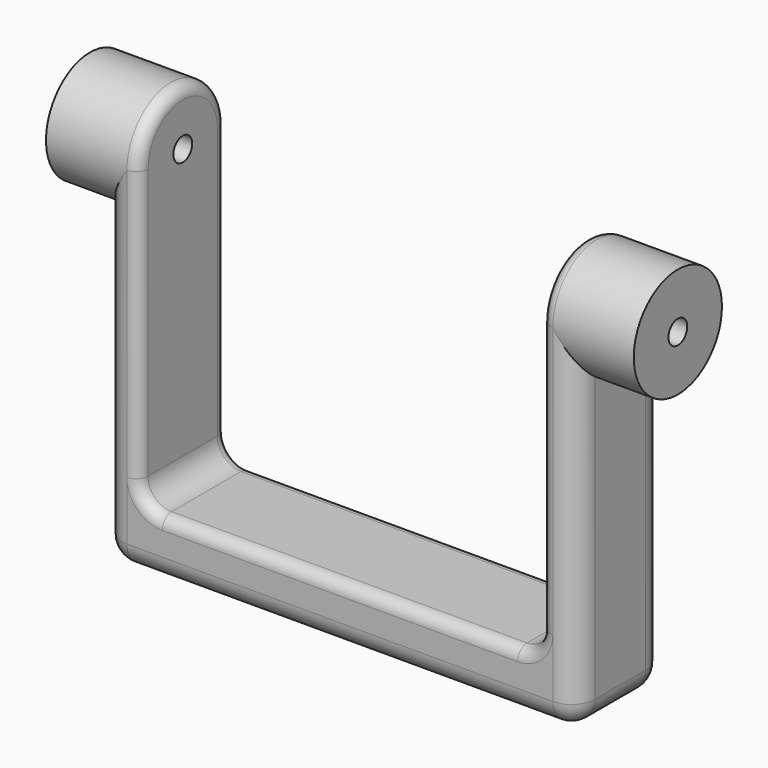
from build123d import *

# Parameters (mm, degrees)
F0_W          = 102.1880283952
F0_H          = 23.8108858466
F1_DEPTH      = 38.1
F2_R          = 11.9054429233
F3_DEPTH      = 63.5
F4_W          = 86.9480283952
F4_H          = 88.2315921943
F5_DEPTH      = 25.4
F6_R          = 2.54
F7_DEPTH      = 63.5
F8_T1_DEPTH   = 127.5880283952
F8_T6_DEPTH   = 101.6
F8_S7_R       = 11.9054429233
F8_T8_DEPTH   = 52
F8_T12_DEPTH  = 101.6
F8_S13_R      = 11.9054429233
F8_T14_DEPTH  = 52
F9_T1_DEPTH   = 127.5880283952
F9_T6_DEPTH   = 101.6
F9_S7_R       = 11.9054429233
F9_T8_DEPTH   = 52
F9_T12_DEPTH  = 101.6
F9_S13_R      = 11.9054429233
F9_T14_DEPTH  = 52
F10_T1_DEPTH  = 13.6508858466
F10_S5_W      = 5.08
F10_S5_H      = 5.08
F10_T6_DEPTH  = 5.08
F10_S11_W     = 5.08
F10_S11_H     = 5.08
F10_T12_DEPTH = 5.08
F10_S17_W     = 5.08
F10_S17_H     = 5.08
F10_T18_DEPTH = 5.08
F10_S23_W     = 5.08
F10_S23_H     = 5.08
F10_T24_DEPTH = 5.08
F11_R         = 5.08
F12_R         = 2.53999


# Not quite as in the source:
# - a fillet or chamfer that OpenCascade refuses, or shapes differently, is made with other operations: its cross-section is extruded or revolved along the edge and cut away or added
# - a fillet or chamfer is up to 0.001 mm smaller than in the source, because OpenCascade refuses the exact size


with BuildPart() as f1:
    # F0 (on Top) → F1 (new body, symmetric)
    with BuildSketch(Plane.XY):
        Rectangle(F0_W, F0_H)
    extrude(amount=F1_DEPTH, both=True)

    # F2 (on Right) → F3 (join, symmetric)
    with BuildSketch(Plane.YZ):
        with Locations((0, 38.1)):
            Circle(F2_R)
    extrude(amount=F3_DEPTH, both=True)

    # F4 (on Front) → F5 (cut, symmetric)
    with BuildSketch(Plane.XZ):
        with Locations((0, 18.7157960971)):
            Rectangle(F4_W, F4_H)
    extrude(amount=F5_DEPTH, both=True, mode=Mode.SUBTRACT)

    # F6 (on Right) → F7 (cut, symmetric)
    with BuildSketch(Plane.YZ):
        with Locations((0, 38.1)):
            Circle(F6_R)
    extrude(amount=F7_DEPTH, both=True, mode=Mode.SUBTRACT)

    # F8: fillet of radius 5.08 on 3 edges, made by hand

    # F8_s2 → F8_t1 (cut)
    with BuildSketch(Plane.YZ.offset(-63.7940141976)):
        with BuildLine():
            ThreePointArc((-6.8254429233, -38.1), (-10.4175453717, -36.6121024484), (-11.9054429233, -33.02))
            Line((-11.9054429233, -33.02), (-11.9054429233, -38.1))
            Line((-11.9054429233, -38.1), (-6.8254429233, -38.1))
        make_face()
    extrude(amount=F8_T1_DEPTH, mode=Mode.SUBTRACT)


with BuildPart() as f8_tool4:
    # F8_s5 → F8_t6 (new body)
    with BuildSketch(Plane.XY.offset(50.8)):
        with BuildLine():
            ThreePointArc((51.0940141976, -6.8254429233), (49.606116646, -10.4175453717), (46.0140141976, -11.9054429233))
            Line((46.0140141976, -11.9054429233), (51.0940141976, -11.9054429233))
            Line((51.0940141976, -11.9054429233), (51.0940141976, -6.8254429233))
        make_face()
    extrude(amount=-F8_T6_DEPTH)

    # F8_s7 → F8_t8 (cut, symmetric)
    with BuildSketch(Plane.YZ.offset(48.6)):
        with Locations((0, 38.1)):
            Circle(F8_S7_R)
    extrude(amount=F8_T8_DEPTH, both=True, mode=Mode.SUBTRACT)


with BuildPart() as f1_1:
    add(f1.part)

    # F8_t3: cut F8_tool4
    add(f8_tool4.part, mode=Mode.SUBTRACT)


with BuildPart() as f8_tool10:
    # F8_s11 → F8_t12 (new body)
    with BuildSketch(Plane.XY.offset(-50.8)):
        with BuildLine():
            ThreePointArc((-51.0940141976, -6.8254429233), (-49.606116646, -10.4175453717), (-46.0140141976, -11.9054429233))
            Line((-46.0140141976, -11.9054429233), (-51.0940141976, -11.9054429233))
            Line((-51.0940141976, -11.9054429233), (-51.0940141976, -6.8254429233))
        make_face()
    extrude(amount=F8_T12_DEPTH)

    # F8_s13 → F8_t14 (cut, symmetric)
    with BuildSketch(Plane.YZ.offset(-48.6)):
        with Locations((0, 38.1)):
            Circle(F8_S13_R)
    extrude(amount=F8_T14_DEPTH, both=True, mode=Mode.SUBTRACT)


with BuildPart() as f1_2:
    add(f1_1.part)

    # F8_t9: cut F8_tool10
    add(f8_tool10.part, mode=Mode.SUBTRACT)

    # F9: fillet of radius 5.08 on 3 edges, made by hand

    # F9_s2 → F9_t1 (cut)
    with BuildSketch(Plane.YZ.offset(-63.7940141976)):
        with BuildLine():
            ThreePointArc((11.9054429233, -33.02), (10.4175453717, -36.6121024484), (6.8254429233, -38.1))
            Line((6.8254429233, -38.1), (11.9054429233, -38.1))
            Line((11.9054429233, -38.1), (11.9054429233, -33.02))
        make_face()
    extrude(amount=F9_T1_DEPTH, mode=Mode.SUBTRACT)


with BuildPart() as f9_tool4:
    # F9_s5 → F9_t6 (new body)
    with BuildSketch(Plane.XY.offset(-50.8)):
        with BuildLine():
            ThreePointArc((-46.0140141976, 11.9054429233), (-49.606116646, 10.4175453717), (-51.0940141976, 6.8254429233))
            Line((-51.0940141976, 6.8254429233), (-51.0940141976, 11.9054429233))
            Line((-51.0940141976, 11.9054429233), (-46.0140141976, 11.9054429233))
        make_face()
    extrude(amount=F9_T6_DEPTH)

    # F9_s7 → F9_t8 (cut, symmetric)
    with BuildSketch(Plane.YZ.offset(-48.6)):
        with Locations((0, 38.1)):
            Circle(F9_S7_R)
    extrude(amount=F9_T8_DEPTH, both=True, mode=Mode.SUBTRACT)


with BuildPart() as f1_3:
    add(f1_2.part)

    # F9_t3: cut F9_tool4
    add(f9_tool4.part, mode=Mode.SUBTRACT)


with BuildPart() as f9_tool10:
    # F9_s11 → F9_t12 (new body)
    with BuildSketch(Plane.XY.offset(50.8)):
        with BuildLine():
            ThreePointArc((46.0140141976, 11.9054429233), (49.606116646, 10.4175453717), (51.0940141976, 6.8254429233))
            Line((51.0940141976, 6.8254429233), (51.0940141976, 11.9054429233))
            Line((51.0940141976, 11.9054429233), (46.0140141976, 11.9054429233))
        make_face()
    extrude(amount=-F9_T12_DEPTH)

    # F9_s13 → F9_t14 (cut, symmetric)
    with BuildSketch(Plane.YZ.offset(48.6)):
        with Locations((0, 38.1)):
            Circle(F9_S13_R)
    extrude(amount=F9_T14_DEPTH, both=True, mode=Mode.SUBTRACT)


with BuildPart() as f1_4:
    add(f1_3.part)

    # F9_t9: cut F9_tool10
    add(f9_tool10.part, mode=Mode.SUBTRACT)

    # F10: fillet of radius 5.08 on 2 edges, made by hand

    # F10_s2 → F10_t1 (cut)
    with BuildSketch(Plane.XZ.offset(-6.8254429233)):
        with BuildLine():
            ThreePointArc((-46.0140141976, -38.1), (-49.606116646, -36.6121024484), (-51.0940141976, -33.02))
            Line((-51.0940141976, -33.02), (-51.0940141976, -38.1))
            Line((-51.0940141976, -38.1), (-46.0140141976, -38.1))
        make_face()
        with BuildLine():
            ThreePointArc((46.0140141976, -38.1), (49.606116646, -36.6121024484), (51.0940141976, -33.02))
            Line((51.0940141976, -33.02), (51.0940141976, -38.1))
            Line((51.0940141976, -38.1), (46.0140141976, -38.1))
        make_face()
    extrude(amount=F10_T1_DEPTH, mode=Mode.SUBTRACT)


with BuildPart() as f10_tool4:
    # F10_s5 → F10_t6 (new body)
    with BuildSketch(Plane.XY.offset(-33.02)):
        with Locations((48.5540141976, -9.3654429233)):
            Rectangle(F10_S5_W, F10_S5_H)
    extrude(amount=-F10_T6_DEPTH)

    # F10_s7 → F10_t8 (revolve, cut)
    with BuildSketch(Plane(origin=(46.0140141976, -6.8254429233, -33.02), x_dir=(-0.7071067812, 0.7071067812, 0), z_dir=(-0.7071067812, -0.7071067812, 0))):
        with BuildLine():
            ThreePointArc((0, -5.08), (5.08, 0), (0, 5.08))
            Line((0, 5.08), (0, -5.08))
        make_face()
    revolve(axis=Axis((46.0140141976, -6.8254429233, -33.02), (0, 0, -1)), mode=Mode.SUBTRACT)


with BuildPart() as f1_5:
    add(f1_4.part)

    # F10_t3: cut F10_tool4
    add(f10_tool4.part, mode=Mode.SUBTRACT)


with BuildPart() as f10_tool10:
    # F10_s11 → F10_t12 (new body)
    with BuildSketch(Plane.XY.offset(-33.02)):
        with Locations((48.5540141976, 9.3654429233)):
            Rectangle(F10_S11_W, F10_S11_H)
    extrude(amount=-F10_T12_DEPTH)

    # F10_s13 → F10_t14 (revolve, cut)
    with BuildSketch(Plane(origin=(46.0140141976, 6.8254429233, -33.02), x_dir=(-0.7071067812, -0.7071067812, 0), z_dir=(0.7071067812, -0.7071067812, 0))):
        with BuildLine():
            ThreePointArc((0, -5.08), (5.08, 0), (0, 5.08))
            Line((0, 5.08), (0, -5.08))
        make_face()
    revolve(axis=Axis((46.0140141976, 6.8254429233, -33.02), (0, 0, -1)), mode=Mode.SUBTRACT)


with BuildPart() as f1_6:
    add(f1_5.part)

    # F10_t9: cut F10_tool10
    add(f10_tool10.part, mode=Mode.SUBTRACT)


with BuildPart() as f10_tool16:
    # F10_s17 → F10_t18 (new body)
    with BuildSketch(Plane.XY.offset(-33.02)):
        with Locations((-48.5540141976, 9.3654429233)):
            Rectangle(F10_S17_W, F10_S17_H)
    extrude(amount=-F10_T18_DEPTH)

    # F10_s19 → F10_t20 (revolve, cut)
    with BuildSketch(Plane(origin=(-46.0140141976, 6.8254429233, -33.02), x_dir=(0.7071067812, -0.7071067812, 0), z_dir=(0.7071067812, 0.7071067812, 0))):
        with BuildLine():
            ThreePointArc((0, -5.08), (5.08, 0), (0, 5.08))
            Line((0, 5.08), (0, -5.08))
        make_face()
    revolve(axis=Axis((-46.0140141976, 6.8254429233, -33.02), (0, 0, -1)), mode=Mode.SUBTRACT)


with BuildPart() as f1_7:
    add(f1_6.part)

    # F10_t15: cut F10_tool16
    add(f10_tool16.part, mode=Mode.SUBTRACT)


with BuildPart() as f10_tool22:
    # F10_s23 → F10_t24 (new body)
    with BuildSketch(Plane.XY.offset(-33.02)):
        with Locations((-48.5540141976, -9.3654429233)):
            Rectangle(F10_S23_W, F10_S23_H)
    extrude(amount=-F10_T24_DEPTH)

    # F10_s25 → F10_t26 (revolve, cut)
    with BuildSketch(Plane(origin=(-46.0140141976, -6.8254429233, -33.02), x_dir=(0.7071067812, 0.7071067812, 0), z_dir=(-0.7071067812, 0.7071067812, 0))):
        with BuildLine():
            ThreePointArc((0, -5.08), (5.08, 0), (0, 5.08))
            Line((0, 5.08), (0, -5.08))
        make_face()
    revolve(axis=Axis((-46.0140141976, -6.8254429233, -33.02), (0, 0, -1)), mode=Mode.SUBTRACT)


with BuildPart() as f1_8:
    add(f1_7.part)

    # F10_t21: cut F10_tool22
    add(f10_tool22.part, mode=Mode.SUBTRACT)

    # F11
    f11_edges = [f1_8.edges().sort_by_distance(p)[0] for p in [
        (-43.474014, 0, -25.4),
        (43.474014, 0, -25.4),
    ]]
    fillet(f11_edges, radius=F11_R)

    # F12 (radius 2.54 in the source; OpenCascade refuses exactly that, so slightly less here)
    f12_edges = [f1_8.edges().sort_by_distance(p)[0] for p in [
        (0, -11.905443, -25.4),
        (-43.474014, -11.905443, 8.89),
        (-41.986117, -11.905443, -23.912102),
        (41.986117, -11.905443, -23.912102),
        (43.474014, -11.905443, 8.89),
    ]]
    fillet(f12_edges, radius=F12_R)


solid = f1_8.part
